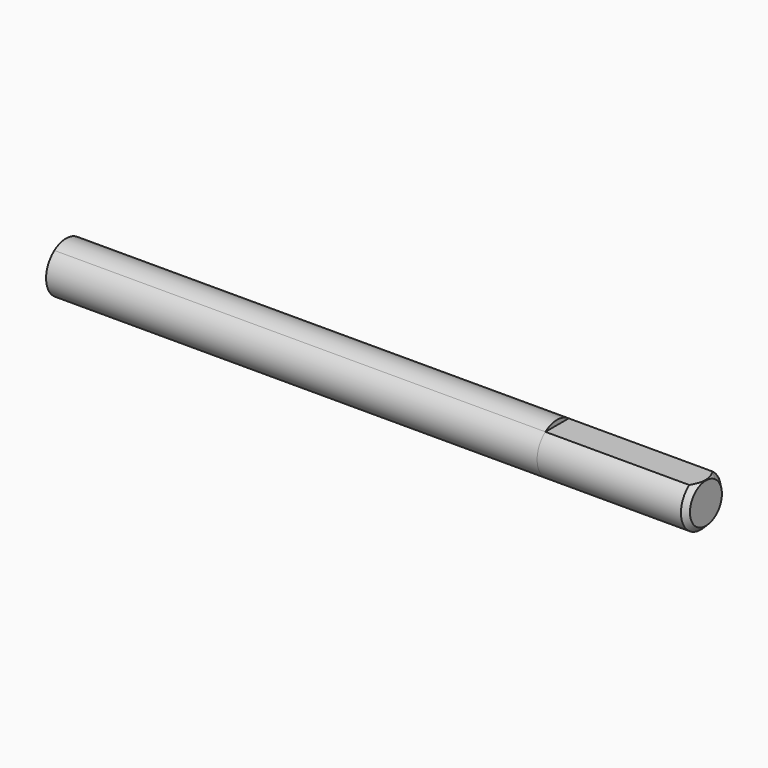
from build123d import *

# Parameters (mm, degrees)
F1_DEPTH    = 49.02
F2_DEPTH    = 14.86
F3_T2_ANGLE = 305.3161054709
F3_T4_ANGLE = 125.133270501


# Not quite as in the source:
# - a fillet or chamfer that OpenCascade refuses, or shapes differently, is made with other operations: its cross-section is extruded or revolved along the edge and cut away or added


with BuildPart() as f1:
    # F0 (on Right) → F1 (new body)
    with BuildSketch(Plane.YZ):
        with BuildLine():
            ThreePointArc((-1.4575321609, 2.025), (-1.1376471902, -2.2205368429), (2.495, 0))
            ThreePointArc((2.495, 0), (2.2205368429, 1.1376471902), (1.4575321609, 2.025))
            Line((1.4575321609, 2.025), (-1.4575321609, 2.025))
        make_face()
        with BuildLine():
            Line((-1.4575321609, 2.025), (1.4575321609, 2.025))
            ThreePointArc((1.4575321609, 2.025), (0, 2.495), (-1.4575321609, 2.025))
        make_face()
    extrude(amount=-F1_DEPTH)

    # F0 (on Right) → F2 (join)
    with BuildSketch(Plane.YZ):
        with BuildLine():
            ThreePointArc((-1.4575321609, 2.025), (-1.1376471902, -2.2205368429), (2.495, 0))
            ThreePointArc((2.495, 0), (2.2205368429, 1.1376471902), (1.4575321609, 2.025))
            Line((1.4575321609, 2.025), (-1.4575321609, 2.025))
        make_face()
    extrude(amount=F2_DEPTH)

    # F3: chamfer of 0.5 on 2 edges, made by hand

    # F3_s1 → F3_t2 (revolve, cut)
    with BuildSketch(Plane(origin=(0, 0, 0), x_dir=(1, 0, 0), z_dir=(0, 0.8159751258, -0.5780870125))):
        with BuildLine():
            Line((14.3458578644, -2.5091421356), (14.8741421356, -1.9808578644))
            Line((14.8741421356, -1.9808578644), (14.8841421356, -1.9808578644))
            ThreePointArc((14.8841421356, -1.9808578644), (14.87, -2.2379289322), (14.87, -2.495))
            Line((14.87, -2.495), (14.86, -2.505))
            ThreePointArc((14.86, -2.505), (14.6029289322, -2.505), (14.3458578644, -2.5191421356))
            Line((14.3458578644, -2.5191421356), (14.3458578644, -2.5091421356))
        make_face()
    revolve(axis=Axis((14.86, 0, 0), (1, 0, 0)), revolution_arc=F3_T2_ANGLE, mode=Mode.SUBTRACT)

    # F3_s3 → F3_t4 (revolve, cut)
    with BuildSketch(Plane.XY):
        with BuildLine():
            Line((14.3458578644, 2.5091421356), (14.8741421356, 1.9808578644))
            Line((14.8741421356, 1.9808578644), (14.8841421356, 1.9808578644))
            ThreePointArc((14.8841421356, 1.9808578644), (14.87, 2.2379289322), (14.87, 2.495))
            Line((14.87, 2.495), (14.86, 2.505))
            ThreePointArc((14.86, 2.505), (14.6029289322, 2.505), (14.3458578644, 2.5191421356))
            Line((14.3458578644, 2.5191421356), (14.3458578644, 2.5091421356))
        make_face()
    revolve(axis=Axis((14.86, 0, 0), (1, 0, 0)), revolution_arc=F3_T4_ANGLE, mode=Mode.SUBTRACT)


solid = f1.part
